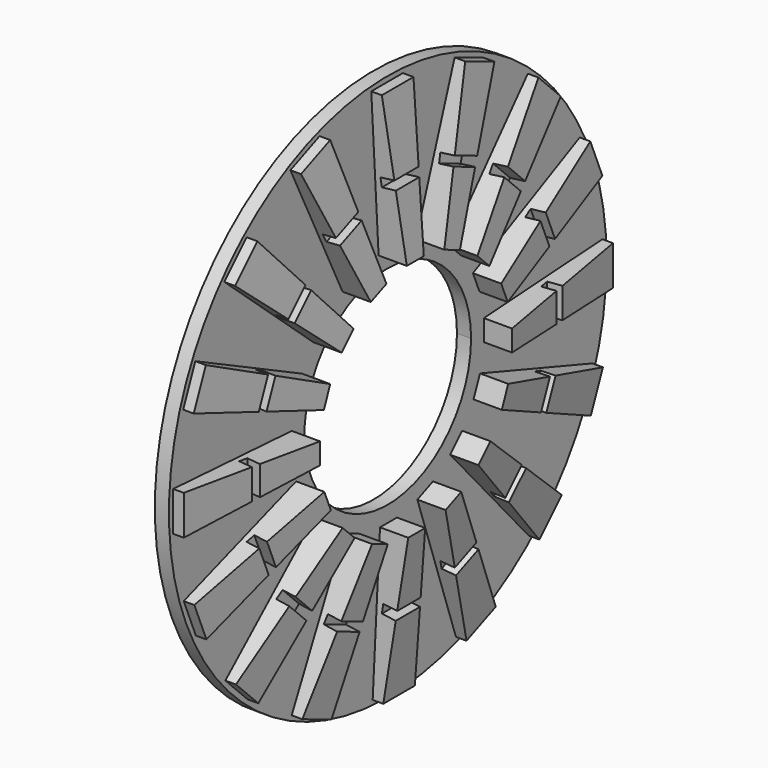
from build123d import *

# Parameters (mm, degrees)
F1_DEPTH    = 6
F2_W        = 6
F2_H        = 1.25
F3_DEPTH    = 2
F4_T1_DEPTH = 132.091103715
F6_COUNT    = 16
F5_R        = 38.75
F7_DEPTH    = 2


# Not quite as in the source:
# - a fillet or chamfer that OpenCascade refuses, or shapes differently, is made with other operations: its cross-section is extruded or revolved along the edge and cut away or added


with BuildPart() as f1:
    # F0 (on Front) → F1 (new body)
    with BuildSketch(Plane.XZ):
        Polygon((0, 21), (0, 0), (6, 0), (3.5, 21), align=None)
    extrude(amount=F1_DEPTH)

    # F2 (on face) → F3 (cut)
    with BuildSketch(Plane(origin=(5.9161542761, 0, 0.7043040805), x_dir=(0, 1, 0), z_dir=(0.9929882742, 0, 0.1182128898))):
        with Locations((-3, 9.2398656526)):
            Rectangle(F2_W, F2_H)
    extrude(amount=-F3_DEPTH, mode=Mode.SUBTRACT)

    # F4: chamfer of 1.5 x 24.25 on 2 edges, made by hand

    # F4_s2 → F4_t1 (cut)
    with BuildSketch(Plane.YZ.offset(-63.0455518575)):
        Polygon((-4.5, 0), (-6, 24.25), (-6, 0), align=None)
        Polygon((-1.5, 0), (0, 24.25), (0, 0), align=None)
    extrude(amount=F4_T1_DEPTH, mode=Mode.SUBTRACT)


with BuildPart() as f6_1:
    # F6: instance of F1
    add(f1.part.rotate(Axis((0, -2.8759991925, -16.9995477528), (1, 0, 0)), 1 * 360 / F6_COUNT))


with BuildPart() as f6_2:
    # F6: instance of F1
    add(f1.part.rotate(Axis((0, -2.8759991925, -16.9995477528), (1, 0, 0)), 2 * 360 / F6_COUNT))


with BuildPart() as f6_3:
    # F6: instance of F1
    add(f1.part.rotate(Axis((0, -2.8759991925, -16.9995477528), (1, 0, 0)), 3 * 360 / F6_COUNT))


with BuildPart() as f6_4:
    # F6: instance of F1
    add(f1.part.rotate(Axis((0, -2.8759991925, -16.9995477528), (1, 0, 0)), 4 * 360 / F6_COUNT))


with BuildPart() as f6_5:
    # F6: instance of F1
    add(f1.part.rotate(Axis((0, -2.8759991925, -16.9995477528), (1, 0, 0)), 5 * 360 / F6_COUNT))


with BuildPart() as f6_6:
    # F6: instance of F1
    add(f1.part.rotate(Axis((0, -2.8759991925, -16.9995477528), (1, 0, 0)), 6 * 360 / F6_COUNT))


with BuildPart() as f6_7:
    # F6: instance of F1
    add(f1.part.rotate(Axis((0, -2.8759991925, -16.9995477528), (1, 0, 0)), 7 * 360 / F6_COUNT))


with BuildPart() as f6_8:
    # F6: instance of F1
    add(f1.part.rotate(Axis((0, -2.8759991925, -16.9995477528), (1, 0, 0)), 8 * 360 / F6_COUNT))


with BuildPart() as f6_9:
    # F6: instance of F1
    add(f1.part.rotate(Axis((0, -2.8759991925, -16.9995477528), (1, 0, 0)), 9 * 360 / F6_COUNT))


with BuildPart() as f6_10:
    # F6: instance of F1
    add(f1.part.rotate(Axis((0, -2.8759991925, -16.9995477528), (1, 0, 0)), 10 * 360 / F6_COUNT))


with BuildPart() as f6_11:
    # F6: instance of F1
    add(f1.part.rotate(Axis((0, -2.8759991925, -16.9995477528), (1, 0, 0)), 11 * 360 / F6_COUNT))


with BuildPart() as f6_12:
    # F6: instance of F1
    add(f1.part.rotate(Axis((0, -2.8759991925, -16.9995477528), (1, 0, 0)), 12 * 360 / F6_COUNT))


with BuildPart() as f6_13:
    # F6: instance of F1
    add(f1.part.rotate(Axis((0, -2.8759991925, -16.9995477528), (1, 0, 0)), 13 * 360 / F6_COUNT))


with BuildPart() as f6_14:
    # F6: instance of F1
    add(f1.part.rotate(Axis((0, -2.8759991925, -16.9995477528), (1, 0, 0)), 14 * 360 / F6_COUNT))


with BuildPart() as f6_15:
    # F6: instance of F1
    add(f1.part.rotate(Axis((0, -2.8759991925, -16.9995477528), (1, 0, 0)), 15 * 360 / F6_COUNT))


with BuildPart() as f1_1:
    add(f1.part)

    add(f6_1.part)  # F7 merges F6_1

    add(f6_2.part)  # F7 merges F6_2

    add(f6_3.part)  # F7 merges F6_3

    add(f6_4.part)  # F7 merges F6_4

    add(f6_5.part)  # F7 merges F6_5

    add(f6_6.part)  # F7 merges F6_6

    add(f6_7.part)  # F7 merges F6_7

    add(f6_8.part)  # F7 merges F6_8

    add(f6_9.part)  # F7 merges F6_9

    add(f6_10.part)  # F7 merges F6_10

    add(f6_11.part)  # F7 merges F6_11

    add(f6_12.part)  # F7 merges F6_12

    add(f6_13.part)  # F7 merges F6_13

    add(f6_14.part)  # F7 merges F6_14

    add(f6_15.part)  # F7 merges F6_15
    # F5 (on Right) → F7 (join)
    with BuildSketch(Plane.YZ):
        with Locations((-2.8759991925, -16.9995477528)):
            Circle(F5_R)
        with BuildLine():
            ThreePointArc((-2.9835881284, -2.2499401438), (7.5157177781, -6.53175341), (11.8740008075, -16.9995477528))
            ThreePointArc((11.8740008075, -16.9995477528), (-13.2677161631, -27.4673420956), (-2.9835881284, -2.2499401438))
        make_face(mode=Mode.SUBTRACT)
    extrude(amount=F7_DEPTH)


solid = f1_1.part
